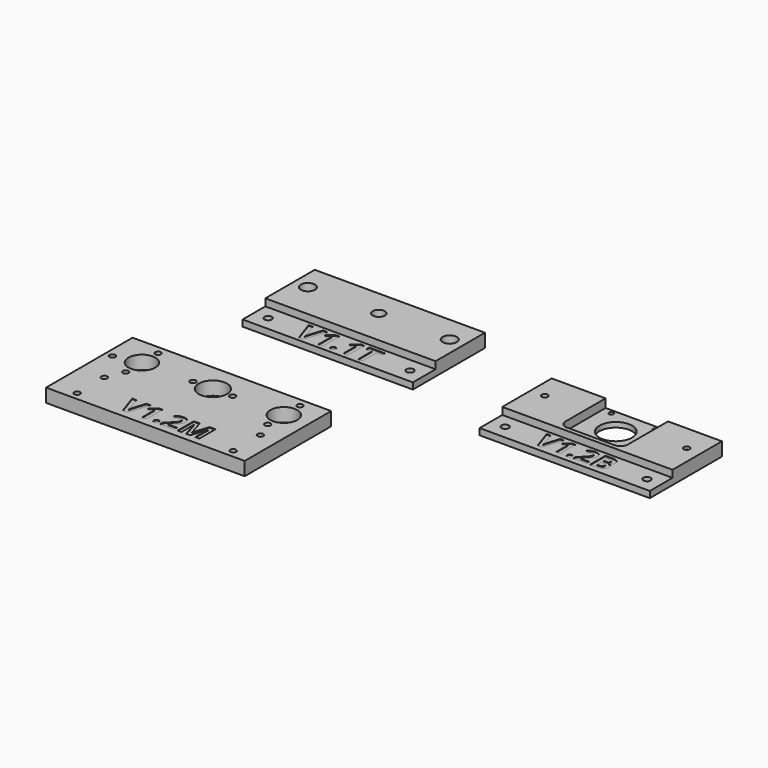
from build123d import *
from build123d import SkipClean  # not in build123d's __all__

# Parameters (mm, degrees)
F0_R          = 2.6
F0_R_2        = 4.25
F0_R_3        = 5
F1_DEPTH      = 4.5
F2_W          = 120
F2_H          = 43.5
F2_R          = 5
F2_R_2        = 4.25
F3_DEPTH      = 5
F4_W          = 135
F4_H          = 76.2
F4_R          = 2.05
F4_R_2        = 9.5
F4_R_3        = 10
F5_DEPTH      = 9.5
F6_W          = 120
F6_H          = 63.5
F6_R          = 2.6
F6_R_2        = 1.6
F6_R_3        = 2.1
F6_R_4        = 11.5
F7_DEPTH      = 4.5
F8_W          = 120
F8_H          = 43.5
F8_R          = 1.6
F8_R_2        = 2.1
F8_R_3        = 11.5
F9_DEPTH      = 5
F10_R         = 5
F11_DEPTH     = 7.5
F13_DEPTH     = 6
F14_TEXT_SIZE = 20.3954321074
F15_DEPTH     = 0.4
F16_TEXT_SIZE = 20.0375704446
F17_DEPTH     = 0.4
F18_TEXT_SIZE = 19.1288638032
F19_DEPTH     = 0.4
F20_DEPTH     = 2
F21_DEPTH     = 5


# Not quite as in the source:
# - after a boolean that leaves OpenCascade's solid faulty, fix() repairs it
# - Text() gives the source's letters only with a copy of the font that has no kerning and outlines rounded to 1/6400 em; it was checked with that copy


with BuildPart() as f1:
    # F0 (on Top) → F1 (new body)
    with BuildSketch(Plane.XY):
        Polygon((-68.7074059993, 0), (-68.7074059993, -10), (51.2925940007, -10), (51.2925940007, 0), (51.2925940007, 10), (-58.7074059993, 10), (-68.7074059993, 10), align=None)
        with BuildLine():
            ThreePointArc((-56.1074059993, 0), (-60.5458836304, -1.8384776311), (-58.7074059993, 2.6))
            ThreePointArc((-58.7074059993, 2.6), (-56.8689283682, 1.8384776311), (-56.1074059993, 0))
        make_face(mode=Mode.SUBTRACT)
        with Locations((41.2925940007, 0)):
            Circle(F0_R, mode=Mode.SUBTRACT)
        Polygon((-68.7074059993, 53.5), (-68.7074059993, 10), (-58.7074059993, 10), (51.2925940007, 10), (51.2925940007, 53.5), align=None)
        with BuildLine():
            ThreePointArc((-53.7074059993, 35), (-55.1718720934, 31.4644660941), (-58.7074059993, 30))
            ThreePointArc((-58.7074059993, 30), (-62.2429399052, 38.5355339059), (-53.7074059993, 35))
        make_face(mode=Mode.SUBTRACT)
        with Locations((-8.7074059993, 35)):
            Circle(F0_R_2, mode=Mode.SUBTRACT)
        with Locations((41.2925940007, 35)):
            Circle(F0_R_3, mode=Mode.SUBTRACT)
    extrude(amount=F1_DEPTH)

    # F2 (on face) → F3 (join)
    with BuildSketch(Plane.XY.offset(4.5)):
        with Locations((-8.7074059993, 31.75)):
            Rectangle(F2_W, F2_H)
        with Locations((-58.7074059993, 35)):
            Circle(F2_R, mode=Mode.SUBTRACT)
        with Locations((-8.7074059993, 35)):
            Circle(F2_R_2, mode=Mode.SUBTRACT)
        with Locations((41.2925940007, 35)):
            Circle(F2_R, mode=Mode.SUBTRACT)
    with SkipClean():  # cleaning this boolean's faces spoils the solid; the shape is the same uncleaned
        extrude(amount=F3_DEPTH)

    # F14 (on face) → F15 (cut)
    with BuildSketch(Plane.XY.offset(4.5)):
        with Locations((-36.1367836595, -7.1206050925)):
            Text('V1.1T', F14_TEXT_SIZE, font='Open Sans', font_style=FontStyle.BOLD, text_align=(TextAlign.LEFT, TextAlign.BOTTOM))
    extrude(amount=-F15_DEPTH, mode=Mode.SUBTRACT)

    add(f1.part.fix(), mode=Mode.REPLACE)


with BuildPart() as f5:
    # F4 (on Top) → F5 (new body)
    with BuildSketch(Plane.XY):
        with Locations((-28.9656567574, -110.3723836184)):
            Rectangle(F4_W, F4_H)
        with Locations((-78.9656567574, -142.9723836184)):
            Circle(F4_R, mode=Mode.SUBTRACT)
        with Locations((-78.9656567574, -118.9723836184)):
            Circle(F4_R, mode=Mode.SUBTRACT)
        with Locations((31.0343432426, -142.9723836184)):
            Circle(F4_R, mode=Mode.SUBTRACT)
        with Locations((31.0343432426, -118.9723836184)):
            Circle(F4_R, mode=Mode.SUBTRACT)
        with Locations((-73.8656567574, -106.5723836184)):
            Circle(F4_R, mode=Mode.SUBTRACT)
        with Locations((-91.4656567574, -96.2723836184)):
            Circle(F4_R, mode=Mode.SUBTRACT)
        with Locations((-73.8656567574, -92.2723836184)):
            Circle(F4_R_2, mode=Mode.SUBTRACT)
        with Locations((-37.8656567574, -92.2723836184)):
            Circle(F4_R, mode=Mode.SUBTRACT)
        with Locations((-73.8656567574, -77.9723836184)):
            Circle(F4_R, mode=Mode.SUBTRACT)
        with Locations((-23.8656567574, -92.2723836184)):
            Circle(F4_R_3, mode=Mode.SUBTRACT)
        with Locations((-9.8656567574, -92.2723836184)):
            Circle(F4_R, mode=Mode.SUBTRACT)
        with Locations((26.1343432426, -106.5723836184)):
            Circle(F4_R, mode=Mode.SUBTRACT)
        with Locations((26.1343432426, -92.2723836184)):
            Circle(F4_R_2, mode=Mode.SUBTRACT)
        with Locations((26.1343432426, -77.9723836184)):
            Circle(F4_R, mode=Mode.SUBTRACT)
    extrude(amount=F5_DEPTH)

    # F16 (on face) → F17 (cut)
    with BuildSketch(Plane.XY.offset(9.5)):
        with Locations((-51.2917710867, -143.3192792386)):
            Text('V1.2M', F16_TEXT_SIZE, font='Open Sans', font_style=FontStyle.BOLD, text_align=(TextAlign.LEFT, TextAlign.BOTTOM))
    extrude(amount=-F17_DEPTH, mode=Mode.SUBTRACT)

    # F21 (add): a face of the model
    f21_faces = [f5.faces().sort_by_distance(p)[0] for p in [
        (38.5343432426, -110.3723836184, 4.75),
    ]]
    extrude(f21_faces, amount=F21_DEPTH)


with BuildPart() as f7:
    # F6 (on Top) → F7 (new body)
    with BuildSketch(Plane.XY):
        with Locations((174.0030223131, 2.1578301936)):
            Rectangle(F6_W, F6_H)
        with Locations((124.0030223131, -19.5921698064)):
            Circle(F6_R, mode=Mode.SUBTRACT)
        with Locations((158.5030223131, -0.0921698064)):
            Circle(F6_R_2, mode=Mode.SUBTRACT)
        with Locations((224.0030223131, -19.5921698064)):
            Circle(F6_R, mode=Mode.SUBTRACT)
        with Locations((189.5030223131, -0.0921698064)):
            Circle(F6_R_2, mode=Mode.SUBTRACT)
        with Locations((124.0030223131, 15.4078301936)):
            Circle(F6_R_3, mode=Mode.SUBTRACT)
        with Locations((158.5030223131, 30.9078301936)):
            Circle(F6_R_2, mode=Mode.SUBTRACT)
        with Locations((174.0030223131, 15.4078301936)):
            Circle(F6_R_4, mode=Mode.SUBTRACT)
        with Locations((224.0030223131, 15.4078301936)):
            Circle(F6_R_3, mode=Mode.SUBTRACT)
        with Locations((189.5030223131, 30.9078301936)):
            Circle(F6_R_2, mode=Mode.SUBTRACT)
    extrude(amount=F7_DEPTH)

    # F8 (on face) → F9 (join)
    with BuildSketch(Plane.XY.offset(4.5)):
        with Locations((174.0030223131, 12.1578301936)):
            Rectangle(F8_W, F8_H)
        with Locations((158.5030223131, -0.0921698064)):
            Circle(F8_R, mode=Mode.SUBTRACT)
        with Locations((189.5030223131, -0.0921698064)):
            Circle(F8_R, mode=Mode.SUBTRACT)
        with Locations((124.0030223131, 15.4078301936)):
            Circle(F8_R_2, mode=Mode.SUBTRACT)
        with Locations((158.5030223131, 30.9078301936)):
            Circle(F8_R, mode=Mode.SUBTRACT)
        with Locations((174.0030223131, 15.4078301936)):
            Circle(F8_R_3, mode=Mode.SUBTRACT)
        with Locations((224.0030223131, 15.4078301936)):
            Circle(F8_R_2, mode=Mode.SUBTRACT)
        with Locations((189.5030223131, 30.9078301936)):
            Circle(F8_R, mode=Mode.SUBTRACT)
    extrude(amount=F9_DEPTH)

    # F10 (on face) → F11 (cut)
    with BuildSketch(Plane.XY):
        with Locations((124.0030223131, 15.4078301936)):
            Circle(F10_R)
        with Locations((224.0030223131, 15.4078301936)):
            Circle(F10_R)
    extrude(amount=F11_DEPTH, mode=Mode.SUBTRACT)

    # F12 (on face) → F13 (cut)
    with BuildSketch(Plane.XY.offset(9.5)):
        with BuildLine():
            Line((196.0030223131, 33.9078301936), (152.0030223131, 33.9078301936))
            Line((152.0030223131, 33.9078301936), (152.0030223131, -1.5921698064))
            ThreePointArc((152.0030223131, -1.5921698064), (153.4674884072, -5.1277037123), (157.0030223131, -6.5921698064))
            Line((157.0030223131, -6.5921698064), (191.0030223131, -6.5921698064))
            ThreePointArc((191.0030223131, -6.5921698064), (194.5385562191, -5.1277037123), (196.0030223131, -1.5921698064))
            Line((196.0030223131, -1.5921698064), (196.0030223131, 33.9078301936))
        make_face()
    extrude(amount=-F13_DEPTH, mode=Mode.SUBTRACT)

    # F18 (on face) → F19 (cut)
    with BuildSketch(Plane.XY.offset(4.5)):
        with Locations((147.2356319427, -25.704331696)):
            Text('V1.2B', F18_TEXT_SIZE, font='Open Sans', font_style=FontStyle.BOLD, text_align=(TextAlign.LEFT, TextAlign.BOTTOM))
    extrude(amount=-F19_DEPTH, mode=Mode.SUBTRACT)

    # F20 (add): a face of the model
    f20_faces = [f7.faces().sort_by_distance(p)[0] for p in [
        (119.1444436694, 15.4078301936, 7.5),
    ]]
    extrude(f20_faces, amount=F20_DEPTH)


solid = Compound([f1.part, f5.part, f7.part])
